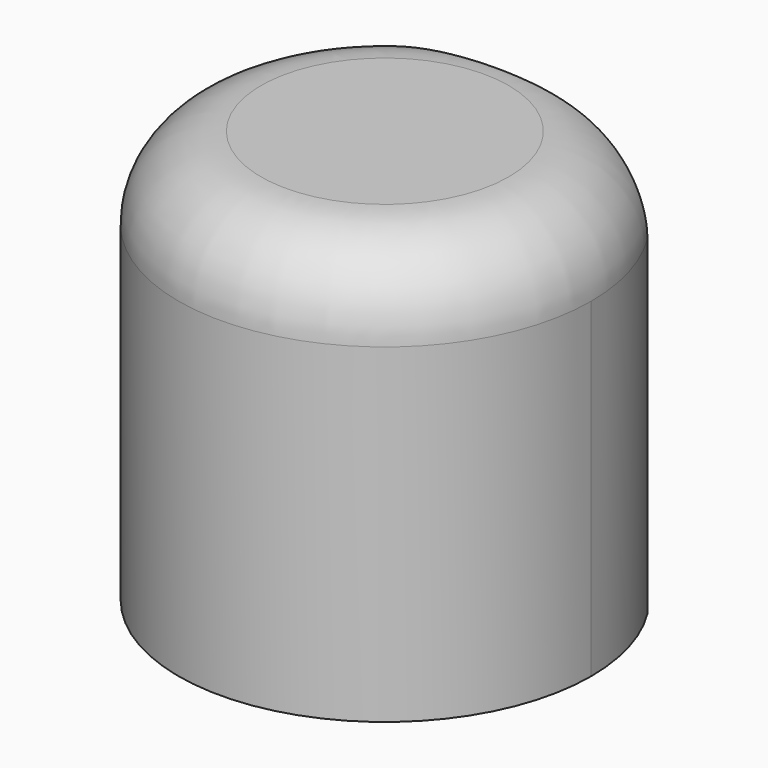
from build123d import *

# Parameters (mm, degrees)
F1_DEPTH    = 25.4
F2_T2_ANGLE = 349.9282786253
F2_T4_ANGLE = 169.6280932898


# Not quite as in the source:
# - a fillet or chamfer that OpenCascade refuses, or shapes differently, is made with other operations: its cross-section is extruded or revolved along the edge and cut away or added


with BuildPart() as f1:
    # F0 (on Top) → F1 (new body)
    with BuildSketch(Plane.XY):
        with BuildLine():
            ThreePointArc((-10.7571298777, 6.7508634111), (-3.512438651, -12.2046210397), (12.7, 0))
            ThreePointArc((12.7, 0), (12.2046210397, 3.512438651), (10.7571298777, 6.7508634111))
            ThreePointArc((10.7571298777, 6.7508634111), (0, 8.6286914647), (-10.7571298777, 6.7508634111))
        make_face()
    extrude(amount=F1_DEPTH)

    # F2: fillet of radius 5.08 on 2 edges, made by hand

    # F2_s1 → F2_t2 (revolve, cut)
    with BuildSketch(Plane(origin=(0, 0, 0), x_dir=(0, 0, 1), z_dir=(0.1748807982, -0.9845896132, 0))):
        with BuildLine():
            ThreePointArc((20.32, -12.7), (23.9121024484, -11.2121024484), (25.4, -7.62))
            Line((25.4, -7.62), (25.5016, -7.62))
            Line((25.5016, -7.62), (25.5016, -12.8016))
            Line((25.5016, -12.8016), (20.32, -12.8016))
            Line((20.32, -12.8016), (20.32, -12.7))
        make_face()
    revolve(axis=Axis((0, 0, 25.4), (0, 0, 1)), revolution_arc=F2_T2_ANGLE, mode=Mode.SUBTRACT)

    # F2_s3 → F2_t4 (revolve, cut)
    with BuildSketch(Plane.XZ):
        with BuildLine():
            ThreePointArc((12.7, 20.32), (11.2121024484, 23.9121024484), (7.62, 25.4))
            Line((7.62, 25.4), (7.62, 25.5016))
            Line((7.62, 25.5016), (12.8016, 25.5016))
            Line((12.8016, 25.5016), (12.8016, 20.32))
            Line((12.8016, 20.32), (12.7, 20.32))
        make_face()
    revolve(axis=Axis((0, 0, 25.4), (0, 0, 1)), revolution_arc=F2_T4_ANGLE, mode=Mode.SUBTRACT)


solid = f1.part
